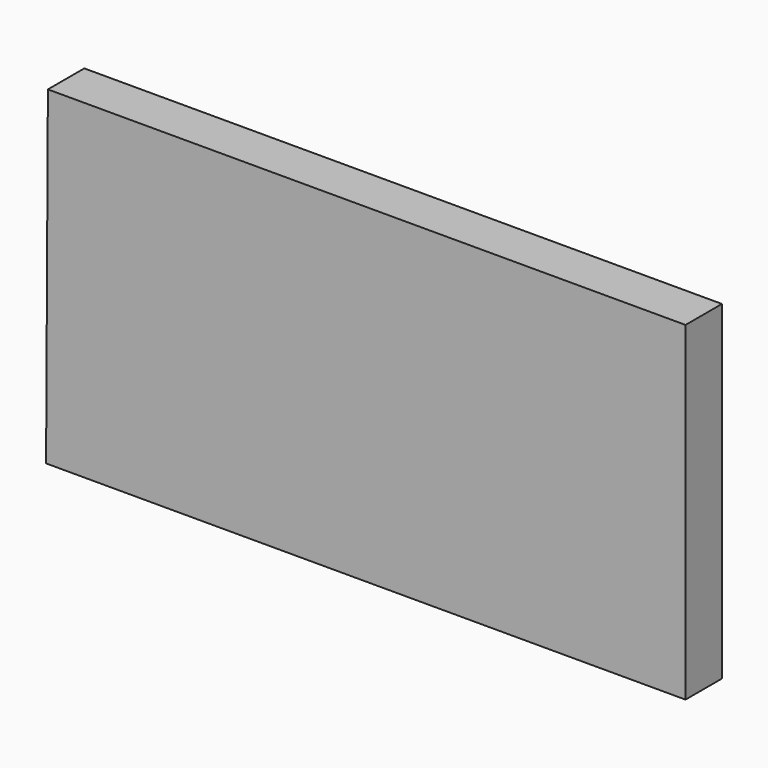
from build123d import *

# Parameters (mm, degrees)
F2_DEPTH = 25.4


# Not quite as in the source:
# - a feature names something its author has since deleted; it is built from what else it names


with BuildPart() as f2:
    # F1 (on face) → F2 (new body)
    with BuildSketch(Plane.XZ):
        Polygon((192.8257749028, -92.4308747053), (192.8257749028, 91.7348861694), (-163.1716638803, 91.7348861694), (-164.1780287027, -92.4308747053), align=None)
    extrude(amount=F2_DEPTH)


solid = f2.part
